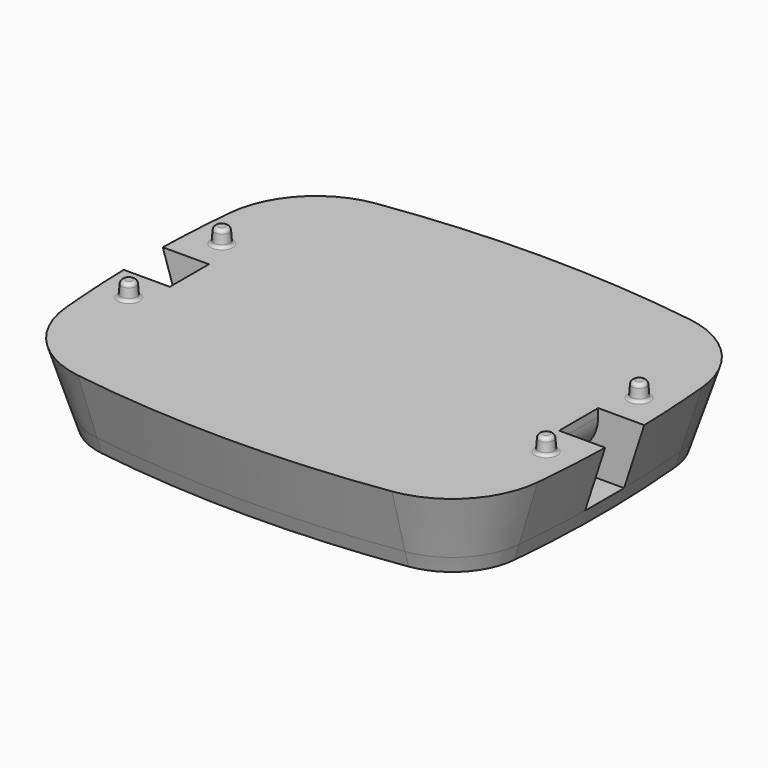
from build123d import *

# Parameters (mm, degrees)
F1_DEPTH    = 7.62
F2_R        = 1.397
F3_DEPTH    = 2.54
F5_R        = 0.635
F6_R        = 0.508
F8_DEPTH    = 2.54
F9_W        = 6.858
F9_H        = 8.001
F10_DEPTH   = 3.81
F11_R       = 6.35
F12_SIZE2   = 3.30199
F12_SIZE    = 10.15999
F12_2_SIZE2 = 3.30199
F12_2_SIZE  = 10.15999
F14_DEPTH   = 2.54
F15_SIZE2   = 2.53999
F15_SIZE    = 0.83819
F16_W       = 38.1
F16_H       = 12.7
F17_DEPTH   = 3.175
F18_W       = 37.084
F18_H       = 11.684
F18_W_2     = 37.592
F18_H_2     = 12.192
F19_DEPTH   = 2.54
F20_W       = 11.1252
F20_H       = 11.1252
F21_DEPTH   = 5.588
F22_R       = 3.556
F23_DEPTH   = 2.541


# Not quite as in the source:
# - a fillet or chamfer that OpenCascade refuses, or shapes differently, is made with other operations: its cross-section is extruded or revolved along the edge and cut away or added
# - a fillet or chamfer is up to 0.001 mm smaller than in the source, because OpenCascade refuses the exact size


with BuildPart() as f1:
    # F0 (on Top) → F1 (new body)
    with BuildSketch(Plane.XY):
        with BuildLine():
            Line((-31.9024, -4.0005), (-39.4519886775, -4.0005))
            ThreePointArc((-39.4519886775, -4.0005), (-39.1897782919, -10.4476626198), (-38.6938068301, -16.8810654862))
            ThreePointArc((-38.6938068301, -16.8810654862), (-34.5656216089, -25.9369938271), (-25.7279005801, -30.5137217362))
            ThreePointArc((-25.7279005801, -30.5137217362), (0, -32.385), (25.7279005801, -30.5137217362))
            ThreePointArc((25.7279005801, -30.5137217362), (34.5656216089, -25.9369938271), (38.6938068301, -16.8810654862))
            ThreePointArc((38.6938068301, -16.8810654862), (39.1897782919, -10.4476626198), (39.4519886775, -4.0005))
            Line((39.4519886775, -4.0005), (31.9024, -4.0005))
            Line((31.9024, -4.0005), (31.9024, 4.0005))
            Line((31.9024, 4.0005), (39.4519886775, 4.0005))
            ThreePointArc((39.4519886775, 4.0005), (39.1897782919, 10.4476626198), (38.6938068301, 16.8810654862))
            ThreePointArc((38.6938068301, 16.8810654862), (34.5656216089, 25.9369938271), (25.7279005801, 30.5137217362))
            ThreePointArc((25.7279005801, 30.5137217362), (0, 32.385), (-25.7279005801, 30.5137217362))
            ThreePointArc((-25.7279005801, 30.5137217362), (-34.5656216089, 25.9369938271), (-38.6938068301, 16.8810654862))
            ThreePointArc((-38.6938068301, 16.8810654862), (-39.1897782919, 10.4476626198), (-39.4519886775, 4.0005))
            Line((-39.4519886775, 4.0005), (-31.9024, 4.0005))
            Line((-31.9024, 4.0005), (-31.9024, -4.0005))
        make_face()
    extrude(amount=-F1_DEPTH)

    # F2 (on Top) → F3 (join)
    with BuildSketch(Plane.XY):
        with Locations((-34.2011, 9.525)):
            Circle(F2_R)
        with Locations((-34.2011, -9.525)):
            Circle(F2_R)
        with Locations((34.2011, 9.525)):
            Circle(F2_R)
        with Locations((34.2011, -9.525)):
            Circle(F2_R)
    extrude(amount=F3_DEPTH)

    # F4: chamfer of 0.254 x 3.556 on 4 edges, made by hand


with BuildPart() as f4_tool2:
    # F4_s3 → F4_t4 (revolve)
    with BuildSketch(Plane.XZ.offset(-9.525)):
        Polygon((-32.8041, -1.016), (-33.0581, 2.54), (-32.8041, 2.54), align=None)
    revolve(axis=Axis((-34.2011, 9.525, 2.54), (0, 0, 1)))

    split(bisect_by=Plane.XY, keep=Keep.TOP)


with BuildPart() as f1_1:
    add(f1.part)

    # F4_t1: cut F4_tool2
    add(f4_tool2.part, mode=Mode.SUBTRACT)


with BuildPart() as f4_tool7:
    # F4_s8 → F4_t9 (revolve)
    with BuildSketch(Plane.XZ.offset(9.525)):
        Polygon((-32.8041, -1.016), (-33.0581, 2.54), (-32.8041, 2.54), align=None)
    revolve(axis=Axis((-34.2011, -9.525, 2.54), (0, 0, 1)))

    split(bisect_by=Plane.XY, keep=Keep.TOP)


with BuildPart() as f1_2:
    add(f1_1.part)

    # F4_t6: cut F4_tool7
    add(f4_tool7.part, mode=Mode.SUBTRACT)


with BuildPart() as f4_tool12:
    # F4_s13 → F4_t14 (revolve)
    with BuildSketch(Plane.XZ.offset(-9.525)):
        Polygon((35.5981, -1.016), (35.3441, 2.54), (35.5981, 2.54), align=None)
    revolve(axis=Axis((34.2011, 9.525, 2.54), (0, 0, 1)))

    split(bisect_by=Plane.XY, keep=Keep.TOP)


with BuildPart() as f1_3:
    add(f1_2.part)

    # F4_t11: cut F4_tool12
    add(f4_tool12.part, mode=Mode.SUBTRACT)


with BuildPart() as f4_tool17:
    # F4_s18 → F4_t19 (revolve)
    with BuildSketch(Plane.XZ.offset(9.525)):
        Polygon((35.5981, -1.016), (35.3441, 2.54), (35.5981, 2.54), align=None)
    revolve(axis=Axis((34.2011, -9.525, 2.54), (0, 0, 1)))

    split(bisect_by=Plane.XY, keep=Keep.TOP)


with BuildPart() as f1_4:
    add(f1_3.part)

    # F4_t16: cut F4_tool17
    add(f4_tool17.part, mode=Mode.SUBTRACT)

    # F5
    f5_edges = [f1_4.edges().sort_by_distance(p)[0] for p in [
        (-35.3441, 9.525, 2.54),
        (-35.3441, -9.525, 2.54),
        (33.0581, 9.525, 2.54),
        (33.0581, -9.525, 2.54),
    ]]
    fillet(f5_edges, radius=F5_R)

    # F6
    f6_edges = [f1_4.edges().sort_by_distance(p)[0] for p in [
        (-35.525529, 9.525, 0),
        (-35.525529, -9.525, 0),
        (32.876671, 9.525, 0),
        (32.876671, -9.525, 0),
    ]]
    fillet(f6_edges, radius=F6_R)

    # F7 (on face) → F8 (join)
    with BuildSketch(Plane(origin=(0, 0, -7.62), x_dir=(1, 0, 0), z_dir=(0, 0, -1))):
        with BuildLine():
            ThreePointArc((-25.7279005801, 30.5137217362), (-34.5656216089, 25.9369938271), (-38.6938068301, 16.8810654862))
            ThreePointArc((-38.6938068301, 16.8810654862), (-39.1897782919, 10.4476626198), (-39.4519886775, 4.0005))
            Line((-39.4519886775, 4.0005), (-10.8712, 4.0005))
            Line((-10.8712, 4.0005), (-10.8712, -4.0005))
            Line((-10.8712, -4.0005), (-39.4519886775, -4.0005))
            ThreePointArc((-39.4519886775, -4.0005), (-39.1897782919, -10.4476626198), (-38.6938068301, -16.8810654862))
            ThreePointArc((-38.6938068301, -16.8810654862), (-34.5656216089, -25.9369938271), (-25.7279005801, -30.5137217362))
            ThreePointArc((-25.7279005801, -30.5137217362), (0, -32.385), (25.7279005801, -30.5137217362))
            ThreePointArc((25.7279005801, -30.5137217362), (34.5656216089, -25.9369938271), (38.6938068301, -16.8810654862))
            ThreePointArc((38.6938068301, -16.8810654862), (39.1897782919, -10.4476626198), (39.4519886775, -4.0005))
            Line((39.4519886775, -4.0005), (10.8712, -4.0005))
            Line((10.8712, -4.0005), (10.8712, 4.0005))
            Line((10.8712, 4.0005), (39.4519886775, 4.0005))
            ThreePointArc((39.4519886775, 4.0005), (39.1897782919, 10.4476626198), (38.6938068301, 16.8810654862))
            ThreePointArc((38.6938068301, 16.8810654862), (34.5656216089, 25.9369938271), (25.7279005801, 30.5137217362))
            ThreePointArc((25.7279005801, 30.5137217362), (0, 32.385), (-25.7279005801, 30.5137217362))
        make_face()
    extrude(amount=F8_DEPTH)

    # F9 (on face) → F10 (cut)
    with BuildSketch(Plane(origin=(0, 0, -7.62), x_dir=(1, 0, 0), z_dir=(0, 0, -1))):
        with Locations((-14.3002, 0)):
            Rectangle(F9_W, F9_H)
        with Locations((14.3002, 0)):
            Rectangle(F9_W, F9_H)
    extrude(amount=-F10_DEPTH, mode=Mode.SUBTRACT)

    # F11
    f11_edges = [f1_4.edges().sort_by_distance(p)[0] for p in [
        (-31.9024, 0, -7.62),
        (31.9024, 0, -7.62),
    ]]
    fillet(f11_edges, radius=F11_R)

    # F12 (size 10.16 and 3.302 in the source; OpenCascade refuses exactly that, so slightly less here)
    f12_edges = [f1_4.edges().sort_by_distance(p)[0] for p in [
        (-34.565622, 25.936994, -10.16),
    ]]
    f12_side = f1_4.faces().sort_by_distance((-34.565622, 25.936994, -5.08))[0]
    chamfer(f12_edges, length=F12_SIZE, length2=F12_SIZE2, reference=f12_side)

    # F12#2 (size 10.16 and 3.302 in the source; OpenCascade refuses exactly that, so slightly less here)
    f12_2_edges = [f1_4.edges().sort_by_distance(p)[0] for p in [
        (-34.565622, -25.936994, -10.16),
    ]]
    f12_2_side = f1_4.faces().sort_by_distance((-34.565622, -25.936994, -5.08))[0]
    chamfer(f12_2_edges, length=F12_2_SIZE, length2=F12_2_SIZE2, reference=f12_2_side)

    # F16 (on face) → F17 (cut)
    with BuildSketch(Plane(origin=(0, 0, -10.16), x_dir=(1, 0, 0), z_dir=(0, 0, -1))):
        with Locations((0, 19.05)):
            Rectangle(F16_W, F16_H)
        with Locations((0, -19.05)):
            Rectangle(F16_W, F16_H)
    extrude(amount=-F17_DEPTH, mode=Mode.SUBTRACT)

    # F20 (on face) → F21 (cut)
    with BuildSketch(Plane(origin=(0, 0, -10.16), x_dir=(1, 0, 0), z_dir=(0, 0, -1))):
        Rectangle(F20_W, F20_H)
    extrude(amount=-F21_DEPTH, mode=Mode.SUBTRACT)


with BuildPart() as f14:
    # F13 (on face) → F14 (new body)
    with BuildSketch(Plane(origin=(0, 0, -10.16), x_dir=(1, 0, 0), z_dir=(0, 0, -1))):
        with BuildLine():
            ThreePointArc((35.4067232747, -16.5675599843), (36.195, 0), (35.4067232747, 16.5675599843))
            ThreePointArc((35.4067232747, 16.5675599843), (32.1729781847, 23.6613705181), (25.2500967122, 27.2464740468))
            ThreePointArc((25.2500967122, 27.2464740468), (0, 29.083), (-25.2500967122, 27.2464740468))
            ThreePointArc((-25.2500967122, 27.2464740468), (-32.1729781847, 23.6613705181), (-35.4067232747, 16.5675599843))
            ThreePointArc((-35.4067232747, 16.5675599843), (-36.195, 0), (-35.4067232747, -16.5675599843))
            ThreePointArc((-35.4067232747, -16.5675599843), (-32.1729781847, -23.6613705181), (-25.2500967122, -27.2464740468))
            ThreePointArc((-25.2500967122, -27.2464740468), (0, -29.083), (25.2500967122, -27.2464740468))
            ThreePointArc((25.2500967122, -27.2464740468), (32.1729781847, -23.6613705181), (35.4067232747, -16.5675599843))
        make_face()
    extrude(amount=F14_DEPTH)

    # F15 (size 0.8382 and 2.54 in the source; OpenCascade refuses exactly that, so slightly less here)
    f15_edges = [f14.edges().sort_by_distance(p)[0] for p in [
        (0, -29.083, -12.7),
    ]]
    f15_side = f14.faces().sort_by_distance((0, 0, -12.7))[0]
    chamfer(f15_edges, length=F15_SIZE, length2=F15_SIZE2, reference=f15_side)

    # F18 (on face) → F19 (join)
    with BuildSketch(Plane.XY.offset(-10.16)):
        with Locations((0, 19.05)):
            Rectangle(F18_W, F18_H)
        with Locations((0, -19.05)):
            Rectangle(F18_W_2, F18_H_2)
    extrude(amount=F19_DEPTH)

    # F22 (on face) → F23 (cut, through all)
    with BuildSketch(Plane.XY.offset(-10.16)):
        Circle(F22_R)
    extrude(amount=-F23_DEPTH, mode=Mode.SUBTRACT)


solid = Compound([f1_4.part, f14.part])
